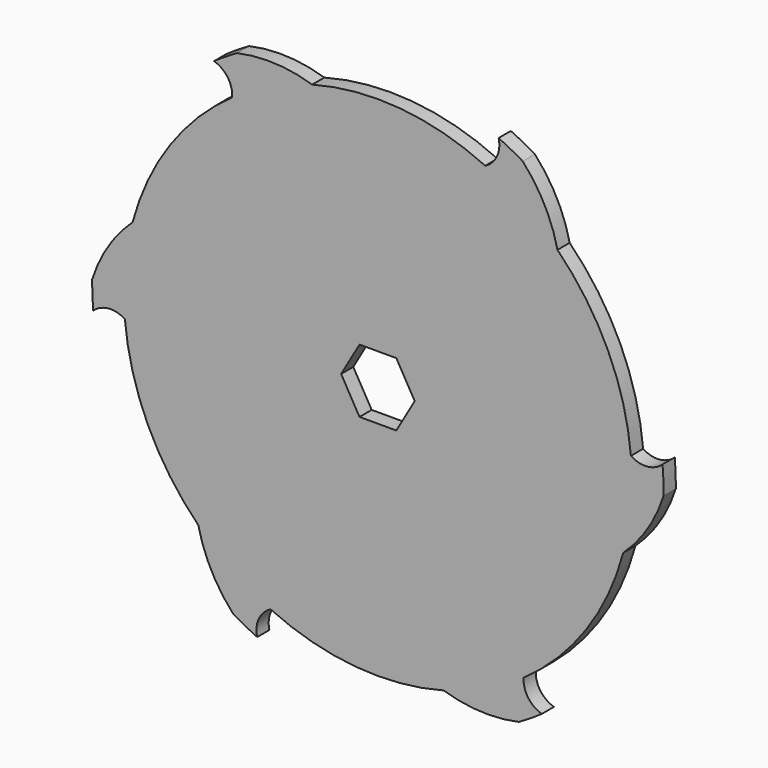
from build123d import *

# Parameters (mm, degrees)
F0_R            = 50.00625
F1_DEPTH        = 1.3335
F3_DEPTH        = 25.4
F3_DEPTH_BACK   = 25.4
F3_COPIES_COUNT = 6


# Not quite as in the source:
# - a pattern or mirror of a feature is missing from the dataset's text; its kind, count and spacing are read off the source's solid


with BuildPart() as f1:
    # F0 (on Front) → F1 (new body, symmetric)
    with BuildSketch(Plane.XZ):
        Circle(F0_R)
        Polygon((-6.4378019116, 0), (-3.2189009558, 5.5753), (3.2189009558, 5.5753), (6.4378019116, 0), (3.2189009558, -5.5753), (-3.2189009558, -5.5753), align=None, mode=Mode.SUBTRACT)
    extrude(amount=F1_DEPTH, both=True)

    # F2 (on Front) → F3 (cut, two sides)
    with BuildSketch(Plane.XZ) as f3_sk:
        with BuildLine():
            ThreePointArc((-11.5045065548, 42.9354029785), (3.8740727651, 44.2808543302), (18.7853817344, 40.2853811338))
            ThreePointArc((18.7853817344, 40.2853811338), (20.8366434022, 42.3941838903), (21.1335544512, 45.3210537755))
            ThreePointArc((21.1335544512, 45.3210537755), (-1.9811990122, 49.9669879974), (-24.6555417703, 43.505508836))
            ThreePointArc((-24.6555417703, 43.505508836), (-18.042450785, 44.0871875941), (-11.5045065548, 42.9354029785))
        make_face()
    f3 = extrude(amount=-F3_DEPTH, mode=Mode.SUBTRACT) + extrude(f3_sk.sketch, amount=F3_DEPTH_BACK, mode=Mode.SUBTRACT)

    # F3_copies: F3 ×6 about axis
    f3_copies_axis = Axis((0, 0, 0), (0, 1, 0))
    for i in range(1, F3_COPIES_COUNT):
        add(f3.rotate(f3_copies_axis, i * 360 / F3_COPIES_COUNT), mode=Mode.SUBTRACT)


solid = f1.part
